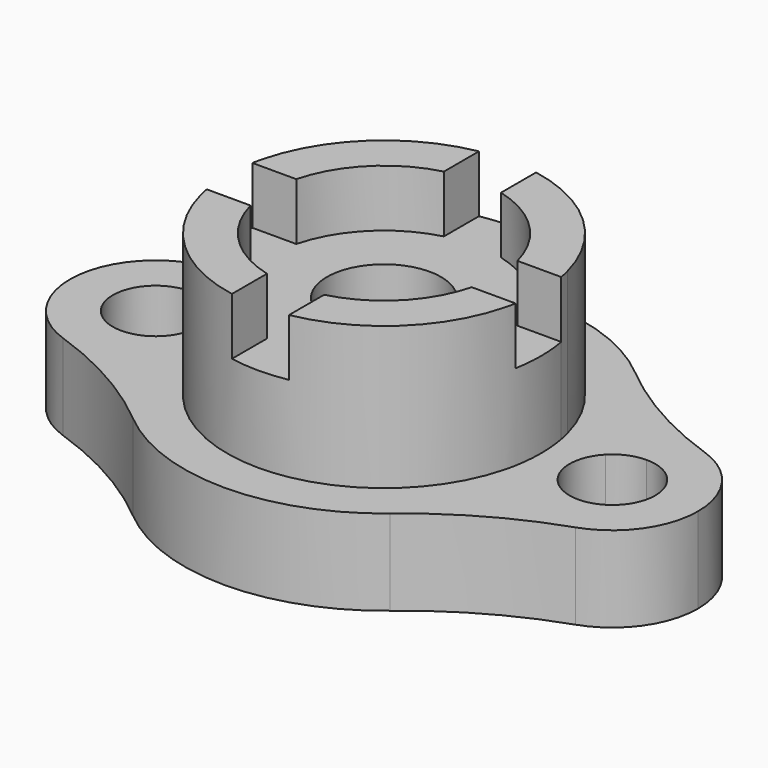
from build123d import *

# Parameters (mm, degrees)
F0_R        = 12.7
F1_DEPTH    = 19.05
F2_DEPTH    = 38.1
F3_DEPTH    = 50.8
F4_T1_DEPTH = 19.05
F5_DEPTH    = 25.4


# Not quite as in the source:
# - a fillet or chamfer that OpenCascade refuses, or shapes differently, is made with other operations: its cross-section is extruded or revolved along the edge and cut away or added


with BuildPart() as f1:
    # F0 (on Top) → F1 (new body)
    with BuildSketch(Plane.XY):
        with BuildLine():
            ThreePointArc((-50.7999117786, -19.0477195084), (-45.869861945, -18.3987278677), (-41.2757240411, -16.4959723838))
            ThreePointArc((-41.2757240411, -16.4959723838), (-42.9000661545, -11.6355843833), (-43.9541916189, -6.620539187))
            ThreePointArc((-43.9541916189, -6.620539187), (-47.0821659857, -8.7672115815), (-50.7999117786, -9.5227195084))
            Line((-50.7999117786, -9.5227195084), (-50.7999117786, -19.0477195084))
        make_face()
        with BuildLine():
            ThreePointArc((33.8339826183, -8.661249632), (23.8448022993, -25.5182489271), (6.35, -34.3428758988))
            ThreePointArc((6.35, -34.3428758988), (0, -34.925), (-6.35, -34.3428758988))
            ThreePointArc((-6.35, -34.3428758988), (-23.8447589032, -25.5182894774), (-33.8339531596, -8.6613647075))
            ThreePointArc((-33.8339531596, -8.6613647075), (-36.9876986012, -13.1173714527), (-41.2757240411, -16.4959723838))
            ThreePointArc((-41.2757240411, -16.4959723838), (2.22821e-05, -44.45), (41.2757405794, -16.495931002))
            ThreePointArc((41.2757405794, -16.495931002), (36.9877138276, -13.1172946041), (33.8339826183, -8.661249632))
        make_face()
        with BuildLine():
            ThreePointArc((6.35, 24.5934442484), (17.9605122421, 17.9605122421), (24.5934442484, 6.35))
            Line((24.5934442484, 6.35), (32.8386816452, 6.35))
            ThreePointArc((32.8386816452, 6.35), (33.2976498796, 7.5235995423), (33.8332048478, 8.6642873181))
            ThreePointArc((33.8332048478, 8.6642873181), (23.8436567211, 25.519319332), (6.35, 34.3428758988))
            Line((6.35, 34.3428758988), (6.35, 24.5934442484))
        make_face()
        with BuildLine():
            ThreePointArc((50.8, 19.0522804916), (45.8690841465, 18.4030568025), (41.2742593566, 16.4996368009))
            ThreePointArc((41.2742593566, 16.4996368009), (42.8990375845, 11.6393760281), (43.9536089212, 6.6244066))
            ThreePointArc((43.9536089212, 6.6244066), (47.0818099956, 8.771584232), (50.8, 9.5272804916))
            Line((50.8, 9.5272804916), (50.8, 19.0522804916))
        make_face()
        with BuildLine():
            ThreePointArc((-43.953597028, 6.6244855122), (-42.8990213005, 11.6394360455), (-41.274242812, 16.4996781876))
            ThreePointArc((-41.274242812, 16.4996781876), (-45.8690358984, 18.4030675143), (-50.7999117786, 19.0522804916))
            Line((-50.7999117786, 19.0522804916), (-50.7999117786, 9.5272804916))
            ThreePointArc((-50.7999117786, 9.5272804916), (-47.0817723125, 8.7716056601), (-43.953597028, 6.6244855122))
        make_face()
        with BuildLine():
            ThreePointArc((-24.5934442484, -6.35), (-25.4, 0), (-24.5934442484, 6.35))
            Line((-24.5934442484, 6.35), (-32.8385934238, 6.35))
            ThreePointArc((-32.8385934238, 6.35), (-32.0240547455, 3.2224812106), (-31.7499117786, 0.0022804916))
            ThreePointArc((-31.7499117786, 0.0022804916), (-32.0244637739, -3.2203042194), (-32.8402059749, -6.35))
            Line((-32.8402059749, -6.35), (-24.5934442484, -6.35))
        make_face()
        with BuildLine():
            ThreePointArc((-34.3428758988, 6.35), (-34.1076619913, 7.5115257095), (-33.8331753774, 8.6644023962))
            ThreePointArc((-33.8331753774, 8.6644023962), (-36.9865207313, 13.1206922771), (-41.274242812, 16.4996781876))
            ThreePointArc((-41.274242812, 16.4996781876), (-42.8990213005, 11.6394360455), (-43.953597028, 6.6244855122))
            ThreePointArc((-43.953597028, 6.6244855122), (-41.9699408557, 3.5740081548), (-41.2749117786, 0.0022804916))
            ThreePointArc((-41.2749117786, 0.0022804916), (-41.9701012053, -3.5698435599), (-43.9541916189, -6.620539187))
            ThreePointArc((-43.9541916189, -6.620539187), (-42.9000661545, -11.6355843833), (-41.2757240411, -16.4959723838))
            ThreePointArc((-41.2757240411, -16.4959723838), (-36.9876986012, -13.1173714527), (-33.8339531596, -8.6613647075))
            ThreePointArc((-33.8339531596, -8.6613647075), (-34.1079991617, -7.5099945529), (-34.3428758988, -6.35))
            ThreePointArc((-34.3428758988, -6.35), (-34.925, 0), (-34.3428758988, 6.35))
        make_face()
        with BuildLine():
            ThreePointArc((-43.9541916189, -6.620539187), (-44.4499999552, 0.0019954336), (-43.953597028, 6.6244855122))
            ThreePointArc((-43.953597028, 6.6244855122), (-47.0817723125, 8.7716056601), (-50.7999117786, 9.5272804916))
            Line((-50.7999117786, 9.5272804916), (-50.7999117786, -9.5227195084))
            ThreePointArc((-50.7999117786, -9.5227195084), (-47.0821659857, -8.7672115815), (-43.9541916189, -6.620539187))
        make_face()
        with BuildLine():
            ThreePointArc((-41.2749117786, 0.0022804916), (-41.9699408557, 3.5740081548), (-43.953597028, 6.6244855122))
            ThreePointArc((-43.953597028, 6.6244855122), (-44.4499999552, 0.0019954336), (-43.9541916189, -6.620539187))
            ThreePointArc((-43.9541916189, -6.620539187), (-41.9701012053, -3.5698435599), (-41.2749117786, 0.0022804916))
        make_face()
        with BuildLine():
            Line((34.3428758988, 6.35), (32.8386816452, 6.35))
            ThreePointArc((32.8386816452, 6.35), (31.7500001536, -0.000138335), (32.8402941963, -6.35))
            Line((32.8402941963, -6.35), (34.3428758988, -6.35))
            ThreePointArc((34.3428758988, -6.35), (34.7791644937, -3.1883133656), (34.925, 0))
            ThreePointArc((34.925, 0), (34.7791644937, 3.1883133656), (34.3428758988, 6.35))
        make_face()
        with BuildLine():
            ThreePointArc((24.5934442484, -6.35), (25.1975542852, -3.2005090291), (25.4, 0))
            ThreePointArc((25.4, 0), (25.1975542852, 3.2005090291), (24.5934442484, 6.35))
            ThreePointArc((24.5934442484, 6.35), (17.9605122421, 17.9605122421), (6.35, 24.5934442484))
            ThreePointArc((6.35, 24.5934442484), (0, 25.4), (-6.35, 24.5934442484))
            ThreePointArc((-6.35, 24.5934442484), (-17.9605122421, 17.9605122421), (-24.5934442484, 6.35))
            ThreePointArc((-24.5934442484, 6.35), (-25.4, 0), (-24.5934442484, -6.35))
            ThreePointArc((-24.5934442484, -6.35), (-17.9605122421, -17.9605122421), (-6.35, -24.5934442484))
            ThreePointArc((-6.35, -24.5934442484), (0, -25.4), (6.35, -24.5934442484))
            ThreePointArc((6.35, -24.5934442484), (17.9605122421, -17.9605122421), (24.5934442484, -6.35))
        make_face()
        Circle(F0_R, mode=Mode.SUBTRACT)
        with BuildLine():
            Line((6.35, -34.3428758988), (6.35, -24.5934442484))
            ThreePointArc((6.35, -24.5934442484), (0, -25.4), (-6.35, -24.5934442484))
            Line((-6.35, -24.5934442484), (-6.35, -34.3428758988))
            ThreePointArc((-6.35, -34.3428758988), (0, -34.925), (6.35, -34.3428758988))
        make_face()
        with BuildLine():
            ThreePointArc((-6.35, 24.5934442484), (0, 25.4), (6.35, 24.5934442484))
            Line((6.35, 24.5934442484), (6.35, 34.3428758988))
            ThreePointArc((6.35, 34.3428758988), (0, 34.925), (-6.35, 34.3428758988))
            Line((-6.35, 34.3428758988), (-6.35, 24.5934442484))
        make_face()
        with BuildLine():
            ThreePointArc((69.85, 0.0022804916), (64.2703841816, 13.4726646732), (50.8, 19.0522804916))
            Line((50.8, 19.0522804916), (50.8, 9.5272804916))
            ThreePointArc((50.8, 9.5272804916), (57.5351920908, 6.7374725824), (60.325, 0.0022804916))
            ThreePointArc((60.325, 0.0022804916), (57.5351920908, -6.7329115992), (50.8, -9.5227195084))
            Line((50.8, -9.5227195084), (50.8, -19.0477195084))
            ThreePointArc((50.8, -19.0477195084), (64.2703841816, -13.46810369), (69.85, 0.0022804916))
        make_face()
        with BuildLine():
            ThreePointArc((-24.5934442484, 6.35), (-17.9605122421, 17.9605122421), (-6.35, 24.5934442484))
            Line((-6.35, 24.5934442484), (-6.35, 34.3428758988))
            ThreePointArc((-6.35, 34.3428758988), (-23.8436133211, 25.5193598821), (-33.8331753774, 8.6644023962))
            ThreePointArc((-33.8331753774, 8.6644023962), (-33.2975871652, 7.5236588976), (-32.8385934238, 6.35))
            Line((-32.8385934238, 6.35), (-24.5934442484, 6.35))
        make_face()
        with BuildLine():
            Line((-6.35, -34.3428758988), (-6.35, -24.5934442484))
            ThreePointArc((-6.35, -24.5934442484), (-17.9605122421, -17.9605122421), (-24.5934442484, -6.35))
            Line((-24.5934442484, -6.35), (-32.8402059749, -6.35))
            ThreePointArc((-32.8402059749, -6.35), (-33.2988800792, -7.5221058258), (-33.8339531596, -8.6613647075))
            ThreePointArc((-33.8339531596, -8.6613647075), (-23.8447589032, -25.5182894774), (-6.35, -34.3428758988))
        make_face()
        with BuildLine():
            Line((-50.7999117786, -9.5227195084), (-50.7999117786, 9.5272804916))
            ThreePointArc((-50.7999117786, 9.5272804916), (-60.3249117786, 0.0022804916), (-50.7999117786, -9.5227195084))
        make_face()
        with BuildLine():
            Line((-50.7999117786, 9.5272804916), (-50.7999117786, 19.0522804916))
            ThreePointArc((-50.7999117786, 19.0522804916), (-69.8499117786, 0.0022804916), (-50.7999117786, -19.0477195084))
            Line((-50.7999117786, -19.0477195084), (-50.7999117786, -9.5227195084))
            ThreePointArc((-50.7999117786, -9.5227195084), (-60.3249117786, 0.0022804916), (-50.7999117786, 9.5272804916))
        make_face()
        with BuildLine():
            ThreePointArc((-31.7499117786, 0.0022804916), (-32.0240547455, 3.2224812106), (-32.8385934238, 6.35))
            Line((-32.8385934238, 6.35), (-34.3428758988, 6.35))
            ThreePointArc((-34.3428758988, 6.35), (-34.925, 0), (-34.3428758988, -6.35))
            Line((-34.3428758988, -6.35), (-32.8402059749, -6.35))
            ThreePointArc((-32.8402059749, -6.35), (-32.0244637739, -3.2203042194), (-31.7499117786, 0.0022804916))
        make_face()
        with BuildLine():
            ThreePointArc((44.45, 0), (44.3257285137, 3.3214893838), (43.9536089212, 6.6244066))
            ThreePointArc((43.9536089212, 6.6244066), (41.2750000096, 0.0018528994), (43.954203504, -6.6204602806))
            ThreePointArc((43.954203504, -6.6204602806), (44.3258775759, -3.319499529), (44.45, 0))
        make_face()
        with BuildLine():
            ThreePointArc((-6.35, 34.3428758988), (0, 34.925), (6.35, 34.3428758988))
            ThreePointArc((6.35, 34.3428758988), (23.8436567211, 25.519319332), (33.8332048478, 8.6642873181))
            ThreePointArc((33.8332048478, 8.6642873181), (36.9865359667, 13.1206154241), (41.2742593566, 16.4996368009))
            ThreePointArc((41.2742593566, 16.4996368009), (2.22855e-05, 44.45), (-41.274242812, 16.4996781876))
            ThreePointArc((-41.274242812, 16.4996781876), (-36.9865207313, 13.1206922771), (-33.8331753774, 8.6644023962))
            ThreePointArc((-33.8331753774, 8.6644023962), (-23.8436133211, 25.5193598821), (-6.35, 34.3428758988))
        make_face()
        with BuildLine():
            ThreePointArc((50.8, 9.5272804916), (47.0818099956, 8.771584232), (43.9536089212, 6.6244066))
            ThreePointArc((43.9536089212, 6.6244066), (44.3257285137, 3.3214893838), (44.45, 0))
            ThreePointArc((44.45, 0), (44.3258775759, -3.319499529), (43.954203504, -6.6204602806))
            ThreePointArc((43.954203504, -6.6204602806), (47.0822036672, -8.7671901554), (50.8, -9.5227195084))
            Line((50.8, -9.5227195084), (50.8, 9.5272804916))
        make_face()
        with BuildLine():
            ThreePointArc((60.325, 0.0022804916), (57.5351920908, 6.7374725824), (50.8, 9.5272804916))
            Line((50.8, 9.5272804916), (50.8, -9.5227195084))
            ThreePointArc((50.8, -9.5227195084), (57.5351920908, -6.7329115992), (60.325, 0.0022804916))
        make_face()
        with BuildLine():
            ThreePointArc((43.954203504, -6.6204602806), (42.9000824312, -11.6355243712), (41.2757405794, -16.495931002))
            ThreePointArc((41.2757405794, -16.495931002), (45.8699101912, -18.3987171574), (50.8, -19.0477195084))
            Line((50.8, -19.0477195084), (50.8, -9.5227195084))
            ThreePointArc((50.8, -9.5227195084), (47.0822036672, -8.7671901554), (43.954203504, -6.6204602806))
        make_face()
        with BuildLine():
            ThreePointArc((24.5934442484, 6.35), (25.1975542852, 3.2005090291), (25.4, 0))
            ThreePointArc((25.4, 0), (25.1975542852, -3.2005090291), (24.5934442484, -6.35))
            Line((24.5934442484, -6.35), (32.8402941963, -6.35))
            ThreePointArc((32.8402941963, -6.35), (31.7500001536, -0.000138335), (32.8386816452, 6.35))
            Line((32.8386816452, 6.35), (24.5934442484, 6.35))
        make_face()
        with BuildLine():
            ThreePointArc((33.8332048478, 8.6642873181), (34.1076747659, 7.5114677036), (34.3428758988, 6.35))
            ThreePointArc((34.3428758988, 6.35), (34.7791644937, 3.1883133656), (34.925, 0))
            ThreePointArc((34.925, 0), (34.7791644937, -3.1883133656), (34.3428758988, -6.35))
            ThreePointArc((34.3428758988, -6.35), (34.1080119331, -7.5099365491), (33.8339826183, -8.661249632))
            ThreePointArc((33.8339826183, -8.661249632), (36.9877138276, -13.1172946041), (41.2757405794, -16.495931002))
            ThreePointArc((41.2757405794, -16.495931002), (42.9000824312, -11.6355243712), (43.954203504, -6.6204602806))
            ThreePointArc((43.954203504, -6.6204602806), (41.2750000096, 0.0018528994), (43.9536089212, 6.6244066))
            ThreePointArc((43.9536089212, 6.6244066), (42.8990375845, 11.6393760281), (41.2742593566, 16.4996368009))
            ThreePointArc((41.2742593566, 16.4996368009), (36.9865359667, 13.1206154241), (33.8332048478, 8.6642873181))
        make_face()
        with BuildLine():
            Line((32.8402941963, -6.35), (24.5934442484, -6.35))
            ThreePointArc((24.5934442484, -6.35), (17.9605122421, -17.9605122421), (6.35, -24.5934442484))
            Line((6.35, -24.5934442484), (6.35, -34.3428758988))
            ThreePointArc((6.35, -34.3428758988), (23.8448022993, -25.5182489271), (33.8339826183, -8.661249632))
            ThreePointArc((33.8339826183, -8.661249632), (33.2989427827, -7.5220464735), (32.8402941963, -6.35))
        make_face()
        with BuildLine():
            ThreePointArc((-33.8339531596, -8.6613647075), (-33.2988800792, -7.5221058258), (-32.8402059749, -6.35))
            Line((-32.8402059749, -6.35), (-34.3428758988, -6.35))
            ThreePointArc((-34.3428758988, -6.35), (-34.1079991617, -7.5099945529), (-33.8339531596, -8.6613647075))
        make_face()
        with BuildLine():
            ThreePointArc((33.8332048478, 8.6642873181), (33.2976498796, 7.5235995423), (32.8386816452, 6.35))
            Line((32.8386816452, 6.35), (34.3428758988, 6.35))
            ThreePointArc((34.3428758988, 6.35), (34.1076747659, 7.5114677036), (33.8332048478, 8.6642873181))
        make_face()
        with BuildLine():
            Line((34.3428758988, -6.35), (32.8402941963, -6.35))
            ThreePointArc((32.8402941963, -6.35), (33.2989427827, -7.5220464735), (33.8339826183, -8.661249632))
            ThreePointArc((33.8339826183, -8.661249632), (34.1080119331, -7.5099365491), (34.3428758988, -6.35))
        make_face()
        with BuildLine():
            Line((-34.3428758988, 6.35), (-32.8385934238, 6.35))
            ThreePointArc((-32.8385934238, 6.35), (-33.2975871652, 7.5236588976), (-33.8331753774, 8.6644023962))
            ThreePointArc((-33.8331753774, 8.6644023962), (-34.1076619913, 7.5115257095), (-34.3428758988, 6.35))
        make_face()
    extrude(amount=F1_DEPTH)

    # F0 (on Top) → F2 (join)
    with BuildSketch(Plane.XY):
        with BuildLine():
            ThreePointArc((-24.5934442484, -6.35), (-25.4, 0), (-24.5934442484, 6.35))
            Line((-24.5934442484, 6.35), (-32.8385934238, 6.35))
            ThreePointArc((-32.8385934238, 6.35), (-32.0240547455, 3.2224812106), (-31.7499117786, 0.0022804916))
            ThreePointArc((-31.7499117786, 0.0022804916), (-32.0244637739, -3.2203042194), (-32.8402059749, -6.35))
            Line((-32.8402059749, -6.35), (-24.5934442484, -6.35))
        make_face()
        with BuildLine():
            ThreePointArc((-31.7499117786, 0.0022804916), (-32.0240547455, 3.2224812106), (-32.8385934238, 6.35))
            Line((-32.8385934238, 6.35), (-34.3428758988, 6.35))
            ThreePointArc((-34.3428758988, 6.35), (-34.925, 0), (-34.3428758988, -6.35))
            Line((-34.3428758988, -6.35), (-32.8402059749, -6.35))
            ThreePointArc((-32.8402059749, -6.35), (-32.0244637739, -3.2203042194), (-31.7499117786, 0.0022804916))
        make_face()
        with BuildLine():
            Line((6.35, -34.3428758988), (6.35, -24.5934442484))
            ThreePointArc((6.35, -24.5934442484), (0, -25.4), (-6.35, -24.5934442484))
            Line((-6.35, -24.5934442484), (-6.35, -34.3428758988))
            ThreePointArc((-6.35, -34.3428758988), (0, -34.925), (6.35, -34.3428758988))
        make_face()
        with BuildLine():
            ThreePointArc((-6.35, 24.5934442484), (0, 25.4), (6.35, 24.5934442484))
            Line((6.35, 24.5934442484), (6.35, 34.3428758988))
            ThreePointArc((6.35, 34.3428758988), (0, 34.925), (-6.35, 34.3428758988))
            Line((-6.35, 34.3428758988), (-6.35, 24.5934442484))
        make_face()
        with BuildLine():
            ThreePointArc((24.5934442484, 6.35), (25.1975542852, 3.2005090291), (25.4, 0))
            ThreePointArc((25.4, 0), (25.1975542852, -3.2005090291), (24.5934442484, -6.35))
            Line((24.5934442484, -6.35), (32.8402941963, -6.35))
            ThreePointArc((32.8402941963, -6.35), (31.7500001536, -0.000138335), (32.8386816452, 6.35))
            Line((32.8386816452, 6.35), (24.5934442484, 6.35))
        make_face()
        with BuildLine():
            Line((34.3428758988, 6.35), (32.8386816452, 6.35))
            ThreePointArc((32.8386816452, 6.35), (31.7500001536, -0.000138335), (32.8402941963, -6.35))
            Line((32.8402941963, -6.35), (34.3428758988, -6.35))
            ThreePointArc((34.3428758988, -6.35), (34.7791644937, -3.1883133656), (34.925, 0))
            ThreePointArc((34.925, 0), (34.7791644937, 3.1883133656), (34.3428758988, 6.35))
        make_face()
        with BuildLine():
            ThreePointArc((24.5934442484, -6.35), (25.1975542852, -3.2005090291), (25.4, 0))
            ThreePointArc((25.4, 0), (25.1975542852, 3.2005090291), (24.5934442484, 6.35))
            ThreePointArc((24.5934442484, 6.35), (17.9605122421, 17.9605122421), (6.35, 24.5934442484))
            ThreePointArc((6.35, 24.5934442484), (0, 25.4), (-6.35, 24.5934442484))
            ThreePointArc((-6.35, 24.5934442484), (-17.9605122421, 17.9605122421), (-24.5934442484, 6.35))
            ThreePointArc((-24.5934442484, 6.35), (-25.4, 0), (-24.5934442484, -6.35))
            ThreePointArc((-24.5934442484, -6.35), (-17.9605122421, -17.9605122421), (-6.35, -24.5934442484))
            ThreePointArc((-6.35, -24.5934442484), (0, -25.4), (6.35, -24.5934442484))
            ThreePointArc((6.35, -24.5934442484), (17.9605122421, -17.9605122421), (24.5934442484, -6.35))
        make_face()
        Circle(F0_R, mode=Mode.SUBTRACT)
        with BuildLine():
            ThreePointArc((33.8332048478, 8.6642873181), (33.2976498796, 7.5235995423), (32.8386816452, 6.35))
            Line((32.8386816452, 6.35), (34.3428758988, 6.35))
            ThreePointArc((34.3428758988, 6.35), (34.1076747659, 7.5114677036), (33.8332048478, 8.6642873181))
        make_face()
        with BuildLine():
            Line((34.3428758988, -6.35), (32.8402941963, -6.35))
            ThreePointArc((32.8402941963, -6.35), (33.2989427827, -7.5220464735), (33.8339826183, -8.661249632))
            ThreePointArc((33.8339826183, -8.661249632), (34.1080119331, -7.5099365491), (34.3428758988, -6.35))
        make_face()
        with BuildLine():
            ThreePointArc((-33.8339531596, -8.6613647075), (-33.2988800792, -7.5221058258), (-32.8402059749, -6.35))
            Line((-32.8402059749, -6.35), (-34.3428758988, -6.35))
            ThreePointArc((-34.3428758988, -6.35), (-34.1079991617, -7.5099945529), (-33.8339531596, -8.6613647075))
        make_face()
        with BuildLine():
            Line((-34.3428758988, 6.35), (-32.8385934238, 6.35))
            ThreePointArc((-32.8385934238, 6.35), (-33.2975871652, 7.5236588976), (-33.8331753774, 8.6644023962))
            ThreePointArc((-33.8331753774, 8.6644023962), (-34.1076619913, 7.5115257095), (-34.3428758988, 6.35))
        make_face()
    extrude(amount=F2_DEPTH)

    # F0 (on Top) → F3 (join)
    with BuildSketch(Plane.XY):
        with BuildLine():
            Line((-6.35, -34.3428758988), (-6.35, -24.5934442484))
            ThreePointArc((-6.35, -24.5934442484), (-17.9605122421, -17.9605122421), (-24.5934442484, -6.35))
            Line((-24.5934442484, -6.35), (-32.8402059749, -6.35))
            ThreePointArc((-32.8402059749, -6.35), (-33.2988800792, -7.5221058258), (-33.8339531596, -8.6613647075))
            ThreePointArc((-33.8339531596, -8.6613647075), (-23.8447589032, -25.5182894774), (-6.35, -34.3428758988))
        make_face()
        with BuildLine():
            Line((32.8402941963, -6.35), (24.5934442484, -6.35))
            ThreePointArc((24.5934442484, -6.35), (17.9605122421, -17.9605122421), (6.35, -24.5934442484))
            Line((6.35, -24.5934442484), (6.35, -34.3428758988))
            ThreePointArc((6.35, -34.3428758988), (23.8448022993, -25.5182489271), (33.8339826183, -8.661249632))
            ThreePointArc((33.8339826183, -8.661249632), (33.2989427827, -7.5220464735), (32.8402941963, -6.35))
        make_face()
        with BuildLine():
            ThreePointArc((6.35, 24.5934442484), (17.9605122421, 17.9605122421), (24.5934442484, 6.35))
            Line((24.5934442484, 6.35), (32.8386816452, 6.35))
            ThreePointArc((32.8386816452, 6.35), (33.2976498796, 7.5235995423), (33.8332048478, 8.6642873181))
            ThreePointArc((33.8332048478, 8.6642873181), (23.8436567211, 25.519319332), (6.35, 34.3428758988))
            Line((6.35, 34.3428758988), (6.35, 24.5934442484))
        make_face()
        with BuildLine():
            ThreePointArc((-24.5934442484, 6.35), (-17.9605122421, 17.9605122421), (-6.35, 24.5934442484))
            Line((-6.35, 24.5934442484), (-6.35, 34.3428758988))
            ThreePointArc((-6.35, 34.3428758988), (-23.8436133211, 25.5193598821), (-33.8331753774, 8.6644023962))
            ThreePointArc((-33.8331753774, 8.6644023962), (-33.2975871652, 7.5236588976), (-32.8385934238, 6.35))
            Line((-32.8385934238, 6.35), (-24.5934442484, 6.35))
        make_face()
        with BuildLine():
            ThreePointArc((-33.8339531596, -8.6613647075), (-33.2988800792, -7.5221058258), (-32.8402059749, -6.35))
            Line((-32.8402059749, -6.35), (-34.3428758988, -6.35))
            ThreePointArc((-34.3428758988, -6.35), (-34.1079991617, -7.5099945529), (-33.8339531596, -8.6613647075))
        make_face()
        with BuildLine():
            Line((-34.3428758988, 6.35), (-32.8385934238, 6.35))
            ThreePointArc((-32.8385934238, 6.35), (-33.2975871652, 7.5236588976), (-33.8331753774, 8.6644023962))
            ThreePointArc((-33.8331753774, 8.6644023962), (-34.1076619913, 7.5115257095), (-34.3428758988, 6.35))
        make_face()
        with BuildLine():
            Line((34.3428758988, -6.35), (32.8402941963, -6.35))
            ThreePointArc((32.8402941963, -6.35), (33.2989427827, -7.5220464735), (33.8339826183, -8.661249632))
            ThreePointArc((33.8339826183, -8.661249632), (34.1080119331, -7.5099365491), (34.3428758988, -6.35))
        make_face()
        with BuildLine():
            ThreePointArc((33.8332048478, 8.6642873181), (33.2976498796, 7.5235995423), (32.8386816452, 6.35))
            Line((32.8386816452, 6.35), (34.3428758988, 6.35))
            ThreePointArc((34.3428758988, 6.35), (34.1076747659, 7.5114677036), (33.8332048478, 8.6642873181))
        make_face()
    extrude(amount=F3_DEPTH)

    # F4: fillet of radius 88.9 on 4 edges, made by hand

    # F4_s2 → F4_t1 (join)
    with BuildSketch(Plane.XY):
        with BuildLine():
            ThreePointArc((28.5765284312, -34.0467990099), (42.0295542971, -24.722587122), (56.9640444636, -18.0228978945))
            ThreePointArc((56.9640444636, -18.0228978945), (48.9545547659, -18.958121189), (41.2757405794, -16.495931002))
            ThreePointArc((41.2757405794, -16.495931002), (36.011708005, -26.0568491296), (28.5765284312, -34.0467990099))
        make_face()
        with BuildLine():
            ThreePointArc((28.5734714877, 34.0493645629), (42.0273344564, 24.7263605674), (56.9624260817, 18.0280122323))
            ThreePointArc((56.9624260817, 18.0280122323), (48.9528524491, 18.9625164059), (41.2742593566, 16.4996368009))
            ThreePointArc((41.2742593566, 16.4996368009), (36.0093683943, 26.0600822685), (28.5734714877, 34.0493645629))
        make_face()
        with BuildLine():
            ThreePointArc((-28.5734917033, 34.0493475985), (-42.0273157024, 24.726354484), (-56.9623641312, 18.0280032511))
            ThreePointArc((-56.9623641312, 18.0280032511), (-48.9528192327, 18.9625217645), (-41.274242812, 16.4996781876))
            ThreePointArc((-41.274242812, 16.4996781876), (-36.0093630649, 26.0600896326), (-28.5734917033, 34.0493475985))
        make_face()
        with BuildLine():
            ThreePointArc((-28.5765486506, -34.0467820392), (-42.0295355464, -24.7225810337), (-56.9639825151, -18.02288891))
            ThreePointArc((-56.9639825151, -18.02288891), (-48.954521553, -18.9581265429), (-41.2757240411, -16.4959723838))
            ThreePointArc((-41.2757240411, -16.4959723838), (-36.0117026803, -26.0568564885), (-28.5765486506, -34.0467820392))
        make_face()
    extrude(amount=F4_T1_DEPTH)

    # F0 (on Top) → F5 (cut)
    with BuildSketch(Plane.XY):
        with BuildLine():
            ThreePointArc((-43.9541916189, -6.620539187), (-44.4499999552, 0.0019954336), (-43.953597028, 6.6244855122))
            ThreePointArc((-43.953597028, 6.6244855122), (-47.0817723125, 8.7716056601), (-50.7999117786, 9.5272804916))
            Line((-50.7999117786, 9.5272804916), (-50.7999117786, -9.5227195084))
            ThreePointArc((-50.7999117786, -9.5227195084), (-47.0821659857, -8.7672115815), (-43.9541916189, -6.620539187))
        make_face()
        with BuildLine():
            ThreePointArc((-41.2749117786, 0.0022804916), (-41.9699408557, 3.5740081548), (-43.953597028, 6.6244855122))
            ThreePointArc((-43.953597028, 6.6244855122), (-44.4499999552, 0.0019954336), (-43.9541916189, -6.620539187))
            ThreePointArc((-43.9541916189, -6.620539187), (-41.9701012053, -3.5698435599), (-41.2749117786, 0.0022804916))
        make_face()
        with BuildLine():
            Line((-50.7999117786, -9.5227195084), (-50.7999117786, 9.5272804916))
            ThreePointArc((-50.7999117786, 9.5272804916), (-60.3249117786, 0.0022804916), (-50.7999117786, -9.5227195084))
        make_face()
        with BuildLine():
            ThreePointArc((44.45, 0), (44.3257285137, 3.3214893838), (43.9536089212, 6.6244066))
            ThreePointArc((43.9536089212, 6.6244066), (41.2750000096, 0.0018528994), (43.954203504, -6.6204602806))
            ThreePointArc((43.954203504, -6.6204602806), (44.3258775759, -3.319499529), (44.45, 0))
        make_face()
        with BuildLine():
            ThreePointArc((50.8, 9.5272804916), (47.0818099956, 8.771584232), (43.9536089212, 6.6244066))
            ThreePointArc((43.9536089212, 6.6244066), (44.3257285137, 3.3214893838), (44.45, 0))
            ThreePointArc((44.45, 0), (44.3258775759, -3.319499529), (43.954203504, -6.6204602806))
            ThreePointArc((43.954203504, -6.6204602806), (47.0822036672, -8.7671901554), (50.8, -9.5227195084))
            Line((50.8, -9.5227195084), (50.8, 9.5272804916))
        make_face()
        with BuildLine():
            ThreePointArc((60.325, 0.0022804916), (57.5351920908, 6.7374725824), (50.8, 9.5272804916))
            Line((50.8, 9.5272804916), (50.8, -9.5227195084))
            ThreePointArc((50.8, -9.5227195084), (57.5351920908, -6.7329115992), (60.325, 0.0022804916))
        make_face()
    extrude(amount=F5_DEPTH, mode=Mode.SUBTRACT)


solid = f1.part
